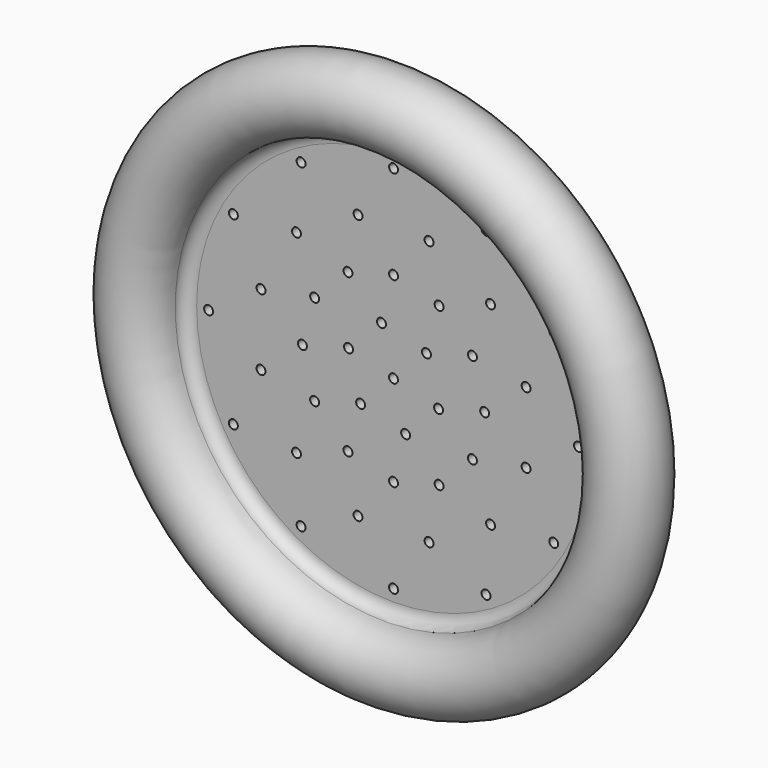
from build123d import *

# Parameters (mm, degrees)
F3_R             = 1.190625
F4_DEPTH         = 6.35
F4_COPIES_COUNT  = 12
F5_R             = 1.190625
F6_DEPTH         = 6.35
F6_COPIES_COUNT  = 12
F7_R             = 1.190625
F8_DEPTH         = 6.35
F8_COPIES_COUNT  = 12
F9_R             = 1.190625
F10_DEPTH        = 6.35
F10_COPIES_COUNT = 6


# Not quite as in the source:
# - a pattern or mirror of a feature is missing from the dataset's text; its kind, count and spacing are read off the source's solid


with BuildPart() as f2:
    # F0 (on Top) → F2 (revolve)
    with BuildSketch(Plane.XY):
        with BuildLine():
            Line((65.0875, 0), (0, 0))
            Line((0, 0), (0, -6.35))
            Line((0, -6.35), (52.3875, -6.35))
            ThreePointArc((52.3875, -6.35), (54.6325640303, -7.2799359697), (55.5625, -9.525))
            ThreePointArc((55.5625, -9.525), (71.8226920908, -16.2601920908), (65.0875, 0))
        make_face()
    revolve(axis=Axis((0, 0, 0), (0, -1, 0)))

    # F3 (on face) → F4 (cut, through all)
    with BuildSketch(Plane.XZ.offset(6.35)):
        with Locations((0, 49.2125)):
            Circle(F3_R)
    f4 = extrude(amount=-F4_DEPTH, mode=Mode.SUBTRACT)

    # F4_copies: F4 ×12 about axis
    f4_copies_axis = Axis((0, 0, 0), (0, 1, 0))
    for i in range(1, F4_COPIES_COUNT):
        add(f4.rotate(f4_copies_axis, i * 360 / F4_COPIES_COUNT), mode=Mode.SUBTRACT)

    # F5 (on face) → F6 (cut, through all)
    with BuildSketch(Plane.XZ.offset(6.35)):
        with Locations((-9.4501303843, 35.2683667324)):
            Circle(F5_R)
    f6 = extrude(amount=-F6_DEPTH, mode=Mode.SUBTRACT)

    # F6_copies: F6 ×12 about axis
    f6_copies_axis = Axis((0, 0, 0), (0, 1, 0))
    for i in range(1, F6_COPIES_COUNT):
        add(f6.rotate(f6_copies_axis, i * 360 / F6_COPIES_COUNT), mode=Mode.SUBTRACT)

    # F7 (on face) → F8 (cut, through all)
    with BuildSketch(Plane.XZ.offset(6.35)):
        with Locations((-20.9970018429, 12.1226246662)):
            Circle(F7_R)
    f8 = extrude(amount=-F8_DEPTH, mode=Mode.SUBTRACT)

    # F8_copies: F8 ×12 about axis
    f8_copies_axis = Axis((0, 0, 0), (0, 1, 0))
    for i in range(1, F8_COPIES_COUNT):
        add(f8.rotate(f8_copies_axis, i * 360 / F8_COPIES_COUNT), mode=Mode.SUBTRACT)

    # F9 (on face) → F10 (cut, through all)
    with BuildSketch(Plane.XZ.offset(6.35)):
        with Locations((-8.7652921912, -8.7652921912)):
            Circle(F9_R)
        Circle(F9_R)
    f10 = extrude(amount=-F10_DEPTH, mode=Mode.SUBTRACT)

    # F10_copies: F10 ×6 about axis
    f10_copies_axis = Axis((0, 0, 0), (0, 1, 0))
    for i in range(1, F10_COPIES_COUNT):
        add(f10.rotate(f10_copies_axis, i * 360 / F10_COPIES_COUNT), mode=Mode.SUBTRACT)


solid = f2.part
